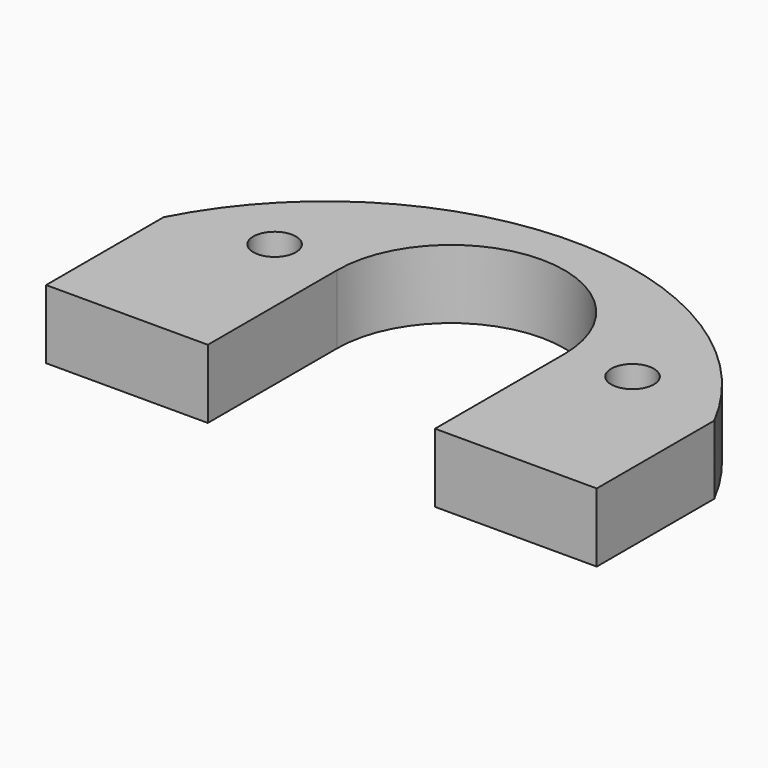
from build123d import *

# Parameters (mm, degrees)
F0_R         = 2.6
F0_R_2       = 2
F0_W         = 7
F0_H         = 10
F1_DEPTH     = 8
F2_DEPTH     = 2.6
F0_R_3       = 6
F3_DEPTH     = 25
F4_R         = 1.65
F5_DEPTH     = 50
F6_DEPTH     = 5
F7_DEPTH     = 2
F9_DEPTH     = 2.6
F10_W        = 6.9695419073
F10_H        = 5.4
F11_DEPTH    = 2.15
F12_R        = 1.65
F13_DEPTH    = 25
F14_R        = 1.55
F15_DEPTH    = 2.7
F16_DEPTH    = 25
F17_R        = 6.99999
F18_W        = 16
F18_H        = 35
F19_DEPTH    = 25
F20_W        = 10
F20_H        = 8
F21_DEPTH    = 16
F22_R        = 5
F23_W        = 31
F23_H        = 60
F24_DEPTH    = 4
F25_W        = 31
F25_H        = 10
F26_DEPTH    = 25
F27_R        = 5
F28_T1_DEPTH = 15
F29_T1_DEPTH = 8
F30_W        = 13.0527611077
F30_H        = 9
F31_DEPTH    = 25
F32_T4_DEPTH = 48
F33_W        = 8
F33_H        = 11
F34_DEPTH    = 8
F35_T4_DEPTH = 8
F36_R        = 2
F37_R        = 2
F39_DEPTH    = 25
F40_DEPTH    = 25
F41_DEPTH    = 7
F42_R        = 2
F43_DEPTH    = 11.75
F44_R        = 2
F45_DEPTH    = 11.75
F47_DEPTH    = 3


# Not quite as in the source:
# - a fillet or chamfer that OpenCascade refuses, or shapes differently, is made with other operations: its cross-section is extruded or revolved along the edge and cut away or added
# - a fillet or chamfer is up to 0.001 mm smaller than in the source, because OpenCascade refuses the exact size


with BuildPart() as f1:
    # F0 (on Top) → F1 (new body)
    with BuildSketch(Plane.XY):
        with BuildLine():
            ThreePointArc((6.1, -34.304502678), (0, -20.5), (-6.1, -34.304502678))
            Line((-6.1, -34.304502678), (-6.1, -28.75))
            ThreePointArc((-6.1, -28.75), (0, -22.65), (6.1, -28.75))
            Line((6.1, -28.75), (6.1, -34.304502678))
        make_face()
        with BuildLine():
            Line((27, 42.5), (-27, 42.5))
            Line((-27, 42.5), (-27, -26.5))
            Line((-27, -26.5), (-20, -26.5))
            Line((-20, -26.5), (-20, -42.5))
            Line((-20, -42.5), (-6.1, -42.5))
            Line((-6.1, -42.5), (-6.1, -34.304502678))
            ThreePointArc((-6.1, -34.304502678), (0, -20.5), (6.1, -34.304502678))
            Line((6.1, -34.304502678), (6.1, -42.5))
            Line((6.1, -42.5), (20, -42.5))
            Line((20, -42.5), (20, -16.5))
            Line((20, -16.5), (27, -16.5))
            Line((27, -16.5), (27, 42.5))
        make_face()
        with Locations((-20.4, -6.1)):
            Circle(F0_R, mode=Mode.SUBTRACT)
        with Locations((-12.5, -13)):
            Circle(F0_R_2, mode=Mode.SUBTRACT)
        with BuildLine():
            add(Edge.make_bspline(
                [(7.5, -13), (7.5, -5.2057713659), (-3.75, -9.102885683), (-15, -13), (-3.75, -16.897114317), (7.5, -20.7942286341), (7.5, -13)],
                knots=[0, 0, 0, 2.0943951024, 2.0943951024, 4.1887902048, 4.1887902048, 6.2831853072, 6.2831853072, 6.2831853072], degree=2, weights=[1, 0.5, 1, 0.5, 1, 0.5, 1]))
        make_face(mode=Mode.SUBTRACT)
        with Locations((20.4, -6.1)):
            Circle(F0_R, mode=Mode.SUBTRACT)
        with Locations((-15.5, 12.5)):
            Rectangle(F0_W, F0_H, mode=Mode.SUBTRACT)
        with Locations((-20.4, 30.9)):
            Circle(F0_R, mode=Mode.SUBTRACT)
        with Locations((15.5, 12.5)):
            Rectangle(F0_W, F0_H, mode=Mode.SUBTRACT)
        with Locations((20.4, 30.9)):
            Circle(F0_R, mode=Mode.SUBTRACT)
    extrude(amount=F1_DEPTH)

    # F0 (on Top) → F2 (cut)
    with BuildSketch(Plane.XY):
        with BuildLine():
            ThreePointArc((6.1, -34.304502678), (0, -20.5), (-6.1, -34.304502678))
            Line((-6.1, -34.304502678), (-6.1, -28.75))
            ThreePointArc((-6.1, -28.75), (0, -22.65), (6.1, -28.75))
            Line((6.1, -28.75), (6.1, -34.304502678))
        make_face()
    extrude(amount=F2_DEPTH, mode=Mode.SUBTRACT)

    # F4 (on Right) → F5 (cut, symmetric)
    with BuildSketch(Plane.YZ):
        with Locations((-36.45, 5.5)):
            Circle(F4_R)
    extrude(amount=F5_DEPTH, both=True, mode=Mode.SUBTRACT)

    # F6 (add): a face of the model
    f6_faces = [f1.faces().sort_by_distance(p)[0] for p in [
        (13.05, -42.5, 4),
    ]]
    extrude(f6_faces, amount=F6_DEPTH)

    # F7 (cut): a face of the model
    f7_faces = [f1.faces().sort_by_distance(p)[0] for p in [
        (-13.05, -42.5, 4),
    ]]
    extrude(f7_faces, amount=-F7_DEPTH, mode=Mode.SUBTRACT)

    # F8 (on face) → F9 (cut, through all)
    with BuildSketch(Plane(origin=(0, 0, 0), x_dir=(1, 0, 0), z_dir=(0, 0, -1))):
        with BuildLine():
            ThreePointArc((6.1, 34.304502678), (7.6937474614, 31.7280446605), (8.25, 28.75))
            Line((8.25, 28.75), (8.25, 47.5))
            Line((8.25, 47.5), (6.1, 47.5))
            Line((6.1, 47.5), (6.1, 34.304502678))
        make_face()
        with BuildLine():
            Line((-8.25, 40.5), (-8.25, 28.75))
            ThreePointArc((-8.25, 28.75), (-7.6937474614, 31.7280446605), (-6.1, 34.304502678))
            Line((-6.1, 34.304502678), (-6.1, 40.5))
            Line((-6.1, 40.5), (-8.25, 40.5))
        make_face()
    extrude(amount=-F9_DEPTH, mode=Mode.SUBTRACT)

    # F10 (on face) → F11 (cut, through all)
    with BuildSketch(Plane(origin=(6.1, 0, 0), x_dir=(0, -1, 0), z_dir=(-1, 0, 0))):
        with Locations((44.0152290463, 5.3)):
            Rectangle(F10_W, F10_H)
    extrude(amount=-F11_DEPTH, mode=Mode.SUBTRACT)

    # F12 (on face) → F13 (cut)
    with BuildSketch(Plane(origin=(8.25, 0, 0), x_dir=(0, -1, 0), z_dir=(-1, 0, 0))):
        with Locations((43.8150316477, 4)):
            Circle(F12_R)
    extrude(amount=-F13_DEPTH, mode=Mode.SUBTRACT)

    # F14 (on face) → F15 (cut)
    with BuildSketch(Plane(origin=(0, 0, 0), x_dir=(1, 0, 0), z_dir=(0, 0, -1))):
        Polygon((-14.6454482672, 25.65), (-11.3545517328, 25.65), (-9.7091034656, 28.5), (-11.3545517328, 31.35), (-14.6454482672, 31.35), (-16.2908965344, 28.5), align=None)
        with Locations((-13, 28.5)):
            Circle(F14_R, mode=Mode.SUBTRACT)
        Polygon((11.3545517328, 31.35), (9.7091034656, 28.5), (11.3545517328, 25.65), (14.6454482672, 25.65), (16.2908965344, 28.5), (14.6454482672, 31.35), align=None)
        with Locations((13, 28.5)):
            Circle(F14_R, mode=Mode.SUBTRACT)
    extrude(amount=-F15_DEPTH, mode=Mode.SUBTRACT)

    # F16 (cut): faces of the model
    f16_faces = [f1.faces().sort_by_distance(p)[0] for p in [
        (-13, -28.5, 0),
        (13, -28.5, 0),
    ]]
    extrude(f16_faces, amount=-F16_DEPTH, mode=Mode.SUBTRACT)

    # F17 (radius 7 in the source; OpenCascade refuses exactly that, so slightly less here)
    f17_edges = [f1.edges().sort_by_distance(p)[0] for p in [
        (27, 42.5, 4),
        (-27, 42.5, 4),
        (-27, -26.5, 4),
        (27, -16.5, 4),
    ]]
    fillet(f17_edges, radius=F17_R)

    # F18 (on face) → F19 (cut)
    with BuildSketch(Plane(origin=(0, 0, 0), x_dir=(1, 0, 0), z_dir=(0, 0, -1))):
        with Locations((0, -15)):
            Rectangle(F18_W, F18_H)
    extrude(amount=-F19_DEPTH, mode=Mode.SUBTRACT)

    # F20 (on face) → F21 (join, through all)
    with BuildSketch(Plane.YZ.offset(-8)):
        with Locations((15.5, 4)):
            Rectangle(F20_W, F20_H)
    extrude(amount=F21_DEPTH)

    # F22
    f22_edges = [f1.edges().sort_by_distance(p)[0] for p in [
        (-8, 10.5, 4),
        (-8, -2.5, 4),
        (8, -2.5, 4),
        (8, 10.5, 4),
        (8, 20.5, 4),
        (-8, 20.5, 4),
        (-8, 32.5, 4),
        (8, 32.5, 4),
    ]]
    fillet(f22_edges, radius=F22_R)

    # F23 (on face) → F24 (cut)
    with BuildSketch(Plane(origin=(0, 0, 0), x_dir=(1, 0, 0), z_dir=(0, 0, -1))):
        with Locations((0, -12.5)):
            Rectangle(F23_W, F23_H)
    extrude(amount=-F24_DEPTH, mode=Mode.SUBTRACT)

    # F25 (on face) → F26 (cut)
    with BuildSketch(Plane(origin=(0, 0, 4), x_dir=(1, 0, 0), z_dir=(0, 0, -1))):
        with Locations((0, 12.5)):
            Rectangle(F25_W, F25_H)
    extrude(amount=-F26_DEPTH, mode=Mode.SUBTRACT)

    # F27
    f27_edges = [f1.edges().sort_by_distance(p)[0] for p in [
        (-19, 12.5, 0),
        (19, 12.5, 0),
    ]]
    fillet(f27_edges, radius=F27_R)

    # F28: fillet of radius 5 on 2 edges, made by hand

    # F28_s2 → F28_t1 (join)
    with BuildSketch(Plane.XZ.offset(-7.5)):
        with BuildLine():
            ThreePointArc((-15.5, 0), (-13.7632981746, 2.8729833462), (-10.6010205144, 4))
            Line((-10.6010205144, 4), (-10.6010205144, 4.1))
            Line((-10.6010205144, 4.1), (-15.5, 4.1))
            Line((-15.5, 4.1), (-15.6, 4))
            ThreePointArc((-15.6, 4), (-15.6, 2), (-15.5979795897, 0.02))
            Line((-15.5979795897, 0.02), (-15.5, 0))
        make_face()
        with BuildLine():
            ThreePointArc((15.5, 0), (13.7632981746, 2.8729833462), (10.6010205144, 4))
            Line((10.6010205144, 4), (10.6010205144, 4.1))
            Line((10.6010205144, 4.1), (15.5, 4.1))
            Line((15.5, 4.1), (15.6, 4))
            ThreePointArc((15.6, 4), (15.6, 2), (15.5979795897, 0.02))
            Line((15.5979795897, 0.02), (15.5, 0))
        make_face()
    extrude(amount=F28_T1_DEPTH)

    # F29: fillet of radius 5 on 4 edges, made by hand

    # F29_s2 → F29_t1 (join)
    with BuildSketch(Plane.XY):
        with BuildLine():
            ThreePointArc((-10.5, -7.5), (-14.0355339059, -8.9644660941), (-15.5, -12.5))
            Line((-15.5, -12.5), (-15.5, -7.5))
            Line((-15.5, -7.5), (-10.5, -7.5))
        make_face()
        with BuildLine():
            ThreePointArc((10.5, -7.5), (14.0355339059, -8.9644660941), (15.5, -12.5))
            Line((15.5, -12.5), (15.5, -7.5))
            Line((15.5, -7.5), (10.5, -7.5))
        make_face()
        with BuildLine():
            ThreePointArc((10.5, -17.5), (14.0355339059, -16.0355339059), (15.5, -12.5))
            Line((15.5, -12.5), (15.5, -17.5))
            Line((15.5, -17.5), (10.5, -17.5))
        make_face()
        with BuildLine():
            ThreePointArc((-15.5, -12.5), (-14.0355339059, -16.0355339059), (-10.5, -17.5))
            Line((-10.5, -17.5), (-15.5, -17.5))
            Line((-15.5, -17.5), (-15.5, -12.5))
        make_face()
    extrude(amount=F29_T1_DEPTH)

    # F30 (on face) → F31 (cut)
    with BuildSketch(Plane(origin=(0, 0, 0), x_dir=(1, 0, 0), z_dir=(0, 0, -1))):
        with Locations((-26.5263805538, 22)):
            Rectangle(F30_W, F30_H)
    extrude(amount=-F31_DEPTH, mode=Mode.SUBTRACT)

    # F32: fillet of radius 8 on 1 edges, made by hand


with BuildPart() as f3:
    # F0 (on Top) → F3 (new body)
    with BuildSketch(Plane.XY):
        with Locations((0, -28.75)):
            Circle(F0_R_3)
    extrude(amount=F3_DEPTH)


with BuildPart() as f32_tool2:
    # F32_s3 → F32_t4 (new body)
    with BuildSketch(Plane.XY.offset(-20)):
        with BuildLine():
            ThreePointArc((-19, -17.5), (-24.6568542495, -15.1568542495), (-27, -9.5))
            Line((-27, -9.5), (-27, -17.5))
            Line((-27, -17.5), (-19, -17.5))
        make_face()
    extrude(amount=F32_T4_DEPTH)

    split(bisect_by=Plane.YZ.offset(-20), keep=Keep.BOTTOM)


with BuildPart() as f1_1:
    add(f1.part)

    # F32_t1: cut F32_tool2
    add(f32_tool2.part, mode=Mode.SUBTRACT)

    # F33 (on Top) → F34 (join, through all)
    with BuildSketch(Plane.XY):
        with Locations((-0.022189036, -12.5)):
            Rectangle(F33_W, F33_H)
    extrude(amount=F34_DEPTH)

    # F35: fillet of radius 5 on 1 edges, made by hand


with BuildPart() as f35_tool2:
    # F35_s3 → F35_t4 (new body)
    with BuildSketch(Plane.YZ.offset(3.977810964)):
        with BuildLine():
            ThreePointArc((-12, 0), (-8.4644660941, 1.4644660941), (-7, 5))
            Line((-7, 5), (-6.9, 5))
            Line((-6.9, 5), (-6.9, -0.1))
            Line((-6.9, -0.1), (-12, -0.1))
            Line((-12, -0.1), (-12, 0))
        make_face()
    extrude(amount=-F35_T4_DEPTH)

    split(bisect_by=Plane.XY.offset(4), keep=Keep.BOTTOM)


with BuildPart() as f1_2:
    add(f1_1.part)

    # F35_t1: cut F35_tool2
    add(f35_tool2.part, mode=Mode.SUBTRACT)

    # F36
    f36_edges = [f1_2.edges().sort_by_distance(p)[0] for p in [
        (3.977811, -7.5, 6),
        (-4.022189, -7.5, 6),
    ]]
    fillet(f36_edges, radius=F36_R)

    # F37
    f37_edges = [f1_2.edges().sort_by_distance(p)[0] for p in [
        (3.977811, -17.5, 4),
        (-4.022189, -17.5, 4),
    ]]
    fillet(f37_edges, radius=F37_R)

    # F38 (on face) → F39 (cut)
    with BuildSketch(Plane.XY.offset(8)):
        with BuildLine():
            ThreePointArc((-22.4970808651, -40.5), (0, -17.6375740767), (22.4970808651, -40.5))
            Line((22.4970808651, -40.5), (37.6332104206, -40.5))
            Line((37.6332104206, -40.5), (37.6332104206, 50.0679649413))
            Line((37.6332104206, 50.0679649413), (-32.9294279218, 50.0679649413))
            Line((-32.9294279218, 50.0679649413), (-32.9294279218, -40.5))
            Line((-32.9294279218, -40.5), (-22.4970808651, -40.5))
        make_face()
    extrude(amount=-F39_DEPTH, mode=Mode.SUBTRACT)

    # F40 (cut): a face of the model
    f40_faces = [f1_2.faces().sort_by_distance(p)[0] for p in [
        (-6.3595128612, -34.625, 2.6),
    ]]
    extrude(f40_faces, amount=-F40_DEPTH, mode=Mode.SUBTRACT)

    # F41 (cut, through all): a face of the model
    f41_faces = [f1_2.faces().sort_by_distance(p)[0] for p in [
        (14.125, -47.5, 4),
    ]]
    extrude(f41_faces, amount=-F41_DEPTH, mode=Mode.SUBTRACT)

    # F42 (on face) → F43 (join, through all)
    with BuildSketch(Plane(origin=(-20, 0, 0), x_dir=(0, -1, 0), z_dir=(-1, 0, 0))):
        with Locations((36.45, 5.5)):
            Circle(F42_R)
    extrude(amount=-F43_DEPTH)

    # F44 (on face) → F45 (join, through all)
    with BuildSketch(Plane.YZ.offset(20)):
        with Locations((-36.45, 5.5)):
            Circle(F44_R)
    extrude(amount=-F45_DEPTH)

    # F47 (cut): a face of the model
    f47_faces = [f1_2.faces().sort_by_distance(p)[0] for p in [
        (0, -18.098300733, 8),
    ]]
    extrude(f47_faces, amount=-F47_DEPTH, mode=Mode.SUBTRACT)


solid = f1_2.part
